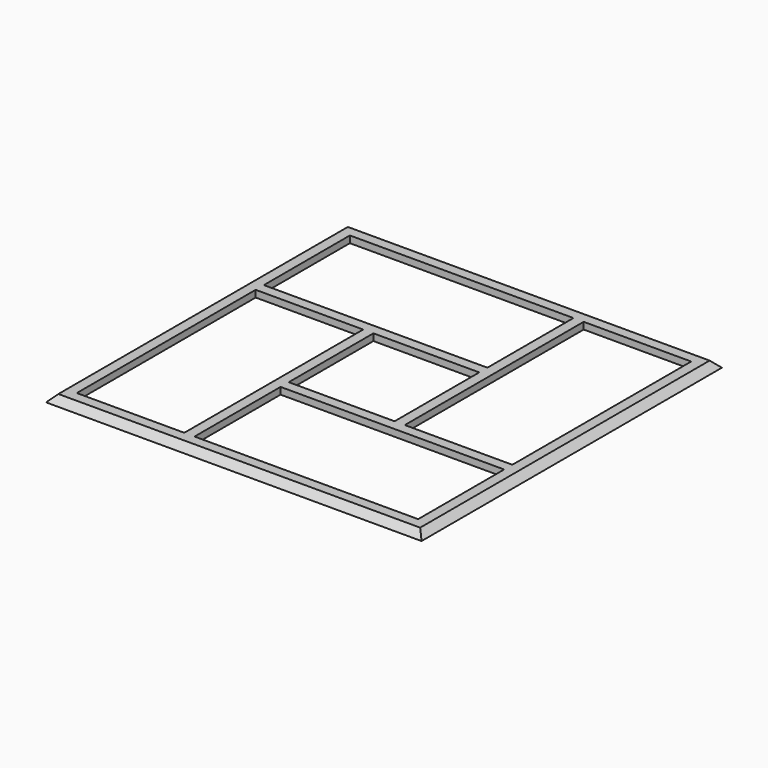
from build123d import *

# Parameters (mm, degrees)
F0_W     = 63
F0_H     = 131
F0_W_2   = 131
F0_H_2   = 63
F0_W_3   = 62
F0_H_3   = 62
F1_DEPTH = 4
F0_W_4   = 4.3501859903
F0_H_4   = 22.087264806
F2_DEPTH = 4
F3_SIZE  = 3.99999
F4_DEPTH = 2


# Not quite as in the source:
# - a fillet or chamfer is up to 0.001 mm smaller than in the source, because OpenCascade refuses the exact size


with BuildPart() as f1:
    # F0 (on Top) → F1 (new body)
    with BuildSketch(Plane.XY):
        Polygon((110, 115.8440702578), (-110, 115.8440702578), (-110, -53.6358393729), (-105.6498140097, -53.6358393729), (-105.6498140097, -75.7231041789), (-110, -75.7231041789), (-110, -104.1559297422), (110, -104.1559297422), align=None)
        with Locations((-68.5, -28.6559297422)):
            Rectangle(F0_W, F0_H, mode=Mode.SUBTRACT)
        with Locations((34.5, -62.6559297422)):
            Rectangle(F0_W_2, F0_H_2, mode=Mode.SUBTRACT)
        with Locations((-34.5, 74.3440702578)):
            Rectangle(F0_W_2, F0_H_2, mode=Mode.SUBTRACT)
        with Locations((0, 5.8440702578)):
            Rectangle(F0_W_3, F0_H_3, mode=Mode.SUBTRACT)
        with Locations((68.5, 40.3440702578)):
            Rectangle(F0_W, F0_H, mode=Mode.SUBTRACT)
    extrude(amount=F1_DEPTH)

    # F0 (on Top) → F2 (join)
    with BuildSketch(Plane.XY):
        Polygon((110, 115.8440702578), (-110, 115.8440702578), (-110, -53.6358393729), (-105.6498140097, -53.6358393729), (-105.6498140097, -75.7231041789), (-110, -75.7231041789), (-110, -104.1559297422), (110, -104.1559297422), align=None)
        with Locations((-68.5, -28.6559297422)):
            Rectangle(F0_W, F0_H, mode=Mode.SUBTRACT)
        with Locations((34.5, -62.6559297422)):
            Rectangle(F0_W_2, F0_H_2, mode=Mode.SUBTRACT)
        with Locations((-34.5, 74.3440702578)):
            Rectangle(F0_W_2, F0_H_2, mode=Mode.SUBTRACT)
        with Locations((0, 5.8440702578)):
            Rectangle(F0_W_3, F0_H_3, mode=Mode.SUBTRACT)
        with Locations((68.5, 40.3440702578)):
            Rectangle(F0_W, F0_H, mode=Mode.SUBTRACT)
        with Locations((-107.8249070048, -64.6794717759)):
            Rectangle(F0_W_4, F0_H_4)
    extrude(amount=F2_DEPTH)

    # F3 (size 4 in the source; OpenCascade refuses exactly that, so slightly less here)
    f3_edges = [f1.edges().sort_by_distance(p)[0] for p in [
        (0, -104.15593, 4),
        (110, 5.84407, 4),
        (-110, 5.84407, 4),
        (0, 115.84407, 4),
    ]]
    chamfer(f3_edges, length=F3_SIZE)

    # F0 (on Top) → F4 (join)
    with BuildSketch(Plane.XY):
        with Locations((-107.8249070048, -64.6794717759)):
            Rectangle(F0_W_4, F0_H_4)
    extrude(amount=-F4_DEPTH)


solid = f1.part
